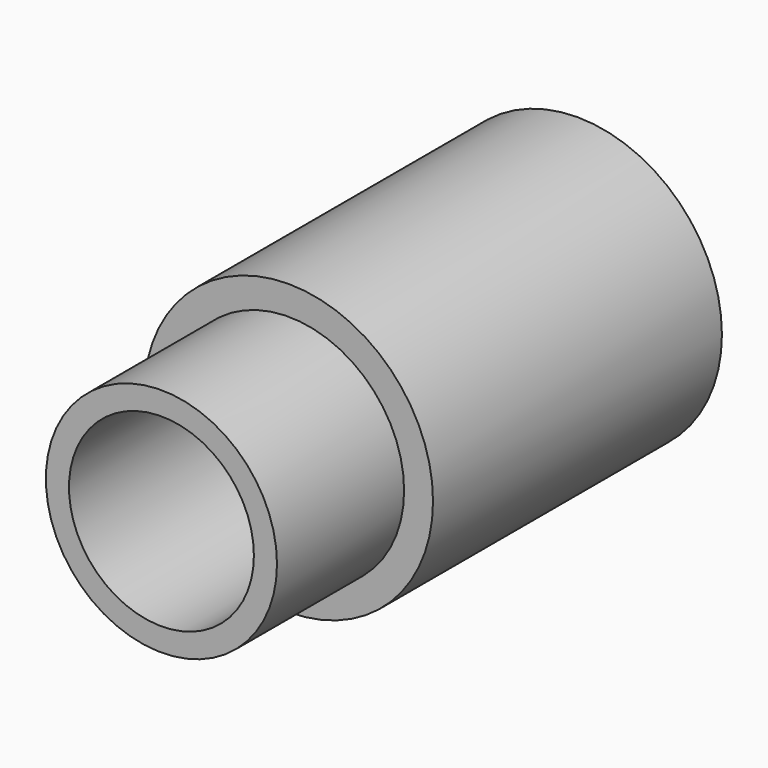
from build123d import *

# Parameters (mm, degrees)
F0_R     = 5
F1_DEPTH = 12.5
F2_R     = 4
F3_DEPTH = 5.5
F5_D     = 6.4


with BuildPart() as f1:
    # F0 (on Front) → F1 (new body)
    with BuildSketch(Plane.XZ):
        Circle(F0_R)
    extrude(amount=F1_DEPTH)

    # F2 (on face) → F3 (join)
    with BuildSketch(Plane.XZ.offset(12.5)):
        Circle(F2_R)
    extrude(amount=F3_DEPTH)

    # F5 (through all)
    with Locations(Plane(origin=(0, 0, 0), x_dir=(-1, 0, 0), z_dir=(0, 1, 0))):
        with Locations((0, 0)):
            Hole(F5_D / 2)


solid = f1.part
